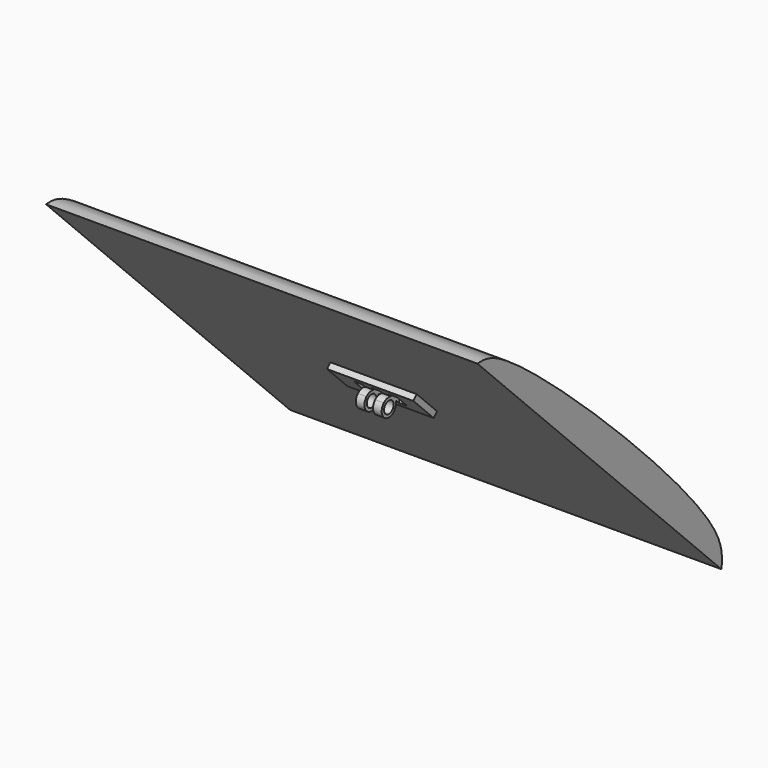
from build123d import *

# Parameters (mm, degrees)
F1_DEPTH  = 457.2
F2_W      = 91.44
F2_H      = 38.1
F3_DEPTH  = 6.35
F4_W      = 45.72
F4_H      = 19.05
F5_DEPTH  = 19.05
F6_W      = 9.144
F6_H      = 19.05
F7_DEPTH  = 25.4
F9_DEPTH  = 27.94
F10_R     = 6.35
F11_DEPTH = 50.8


with BuildPart() as f1:
    # F0 (on Right) → F1 (new body)
    with BuildSketch(Plane.YZ):
        with BuildLine():
            add(Edge.make_bspline(
                [(0, 0), (7.9206921486, 0.4964849945), (41.788781698, 2.6194053072), (328.8937583875, -268.1300359687), (324.4514783657, -311.8504178384), (323.2892203585, -323.2892203585)],
                knots=[0, 0, 0, 0, 0.1839351844, 0.786488501, 1, 1, 1, 1], degree=3))
            Line((0, 0), (323.2892203585, -323.2892203585))
        make_face()
    extrude(amount=F1_DEPTH)

    # F2 (on face) → F3 (join)
    with BuildSketch(Plane(origin=(0, 0, 0), x_dir=(1, 0, 0), z_dir=(0, -0.7071067812, -0.7071067812))):
        with Locations((228.6, -228.6)):
            Rectangle(F2_W, F2_H)
    extrude(amount=F3_DEPTH)

    # F4 (on face) → F5 (join)
    with BuildSketch(Plane(origin=(0, -4.4901280605, -4.4901280605), x_dir=(1, 0, 0), z_dir=(0, -0.7071067812, -0.7071067812))):
        with Locations((228.6, -228.6)):
            Rectangle(F4_W, F4_H)
    extrude(amount=F5_DEPTH)

    # F6 (on face) → F7 (cut)
    with BuildSketch(Plane(origin=(0, -17.9605122421, -17.9605122421), x_dir=(1, 0, 0), z_dir=(0, -0.7071067812, -0.7071067812))):
        with Locations((210.312, -228.6)):
            Rectangle(F6_W, F6_H)
        with Locations((228.6, -228.6)):
            Rectangle(F6_W, F6_H)
        with Locations((246.888, -228.6)):
            Rectangle(F6_W, F6_H)
    extrude(amount=-F7_DEPTH, mode=Mode.SUBTRACT)

    # F8 (on face) → F9 (cut)
    with BuildSketch(Plane.YZ.offset(242.316)):
        with BuildLine():
            ThreePointArc((144.492320988, -165.3265151889), (148.8943740988, -162.8268771513), (153.9554431224, -162.9356992435))
            Line((153.9554431224, -162.9356992435), (150.4192900279, -159.399546149))
            Line((150.4192900279, -159.399546149), (144.492320988, -165.3265151889))
        make_face()
        with BuildLine():
            ThreePointArc((160.353521115, -169.3337772361), (160.6522372537, -170.683230139), (160.7525130788, -172.0617072797))
            ThreePointArc((160.7525130788, -172.0617072797), (160.027465626, -175.706766973), (157.9627051696, -178.7968993705))
            Line((157.9627051696, -178.7968993705), (163.8896742095, -172.8699303306))
            Line((163.8896742095, -172.8699303306), (160.353521115, -169.3337772361))
        make_face()
        with BuildLine():
            Line((150.4192900279, -186.3403145122), (157.9627051696, -178.7968993705))
            ThreePointArc((157.9627051696, -178.7968993705), (144.492320988, -178.7968993705), (144.492320988, -165.3265151889))
            Line((144.492320988, -165.3265151889), (136.9489058463, -172.8699303306))
            Line((136.9489058463, -172.8699303306), (150.4192900279, -186.3403145122))
        make_face()
    extrude(amount=-F9_DEPTH, mode=Mode.SUBTRACT)

    # F10 (on face) → F11 (cut)
    with BuildSketch(Plane(origin=(214.884, 0, 0), x_dir=(0, -1, 0), z_dir=(-1, 0, 0))):
        with Locations((-151.2275130788, -172.0617072797)):
            Circle(F10_R)
    extrude(amount=-F11_DEPTH, mode=Mode.SUBTRACT)


solid = f1.part
